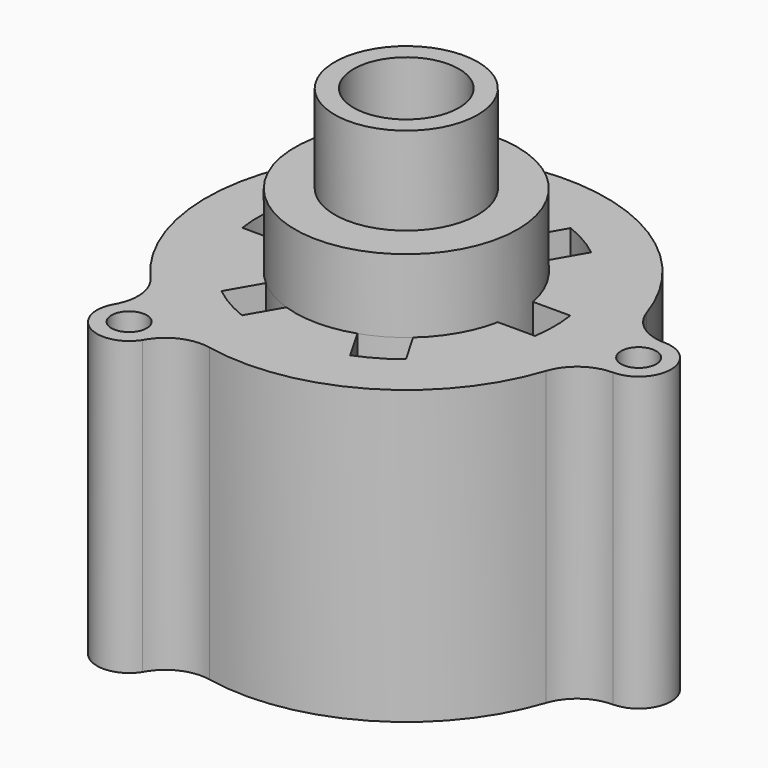
from build123d import *
from build123d import SkipClean  # not in build123d's __all__

# Parameters (mm, degrees)
F0_R      = 7.588
F0_R_2    = 1.105
F1_DEPTH  = 1.32
F2_R      = 7.588
F2_R_2    = 5.588
F3_DEPTH  = 5
F4_R      = 8.638
F4_R_2    = 5.588
F5_DEPTH  = 10
F6_R      = 1.2
F6_R_2    = 3.588
F7_DEPTH  = 2
F8_R      = 1.2
F8_R_2    = 12.138
F9_DEPTH  = 17.92
F10_R     = 4.875
F10_R_2   = 3.588
F11_DEPTH = 11
F13_DEPTH = 2
F15_R     = 7.588
F15_R_2   = 4.875
F16_DEPTH = 5
F17_R     = 5.588
F17_R_2   = 3.588
F18_DEPTH = 13
F19_R     = 7.588
F20_DEPTH = 1.32


# Not quite as in the source:
# - after a boolean that leaves OpenCascade's solid faulty, fix() repairs it


with BuildPart() as f1:
    # F0 (on Top) → F1 (new body)
    with BuildSketch(Plane.XY):
        Circle(F0_R)
        with BuildLine():
            ThreePointArc((-0.0759227724, -1.9785438415), (0.99, -1.7147302995), (1.7514306154, -0.9235208711))
            ThreePointArc((1.7514306154, -0.9235208711), (2.7984444548, -0.5994652894), (3.1225000365, -1.6464791289))
            ThreePointArc((3.1225000365, -1.6464791289), (1.765, -3.0570696754), (-0.1353572659, -3.5274039194))
            ThreePointArc((-0.1353572659, -3.5274039194), (-0.8800700581, -2.7232566337), (-0.0759227724, -1.9785438415))
        make_face(mode=Mode.SUBTRACT)
        with BuildLine():
            ThreePointArc((-2.9871427707, 1.8809247905), (-1.9183743967, 2.1237913442), (-1.675507843, 1.0550229703))
            ThreePointArc((-1.675507843, 1.0550229703), (-1.98, 0), (-1.675507843, -1.0550229703))
            ThreePointArc((-1.675507843, -1.0550229703), (-1.9183743967, -2.1237913442), (-2.9871427707, -1.8809247905))
            ThreePointArc((-2.9871427707, -1.8809247905), (-3.53, 0), (-2.9871427707, 1.8809247905))
        make_face(mode=Mode.SUBTRACT)
        Circle(F0_R_2, mode=Mode.SUBTRACT)
        with BuildLine():
            ThreePointArc((3.1225000365, 1.6464791289), (2.7984444548, 0.5994652894), (1.7514306154, 0.9235208711))
            ThreePointArc((1.7514306154, 0.9235208711), (0.99, 1.7147302995), (-0.0759227724, 1.9785438415))
            ThreePointArc((-0.0759227724, 1.9785438415), (-0.8800700581, 2.7232566337), (-0.1353572659, 3.5274039194))
            ThreePointArc((-0.1353572659, 3.5274039194), (1.765, 3.0570696754), (3.1225000365, 1.6464791289))
        make_face(mode=Mode.SUBTRACT)
    extrude(amount=F1_DEPTH)

    # F2 (on face) → F3 (join)
    with BuildSketch(Plane.XY.offset(1.32)):
        Circle(F2_R)
        Circle(F2_R_2, mode=Mode.SUBTRACT)
    extrude(amount=F3_DEPTH)

    # F4 (on face) → F5 (join)
    with BuildSketch(Plane.XY.offset(6.32)):
        Circle(F4_R)
        Circle(F4_R_2, mode=Mode.SUBTRACT)
    extrude(amount=F5_DEPTH)

    # F6 (on face) → F7 (join)
    with BuildSketch(Plane.XY.offset(16.32)):
        with BuildLine():
            ThreePointArc((-9.7367268731, 12.4452239819), (-9.4590741999, 10.5147410615), (-10.4092493603, 8.8115022416))
            ThreePointArc((-10.4092493603, 8.8115022416), (-13.6367061296, -0.1878561577), (-10.1625749103, -9.0948950073))
            ThreePointArc((-10.1625749103, -9.0948950073), (-9.4051511551, -10.8523580323), (-9.8453718266, -12.7147685106))
            ThreePointArc((-9.8453718266, -12.7147685106), (-9.001992595, -15.6331871577), (-6.0474096405, -14.9268618126))
            ThreePointArc((-6.0474096405, -14.9268618126), (-4.651452375, -13.5895530665), (-2.731783232, -13.361601864))
            ThreePointArc((-2.731783232, -13.361601864), (6.8311346088, -11.8038402208), (12.9462201401, -4.2884062405))
            ThreePointArc((12.9462201401, -4.2884062405), (14.0544760036, -2.7766870908), (15.838, -2.2))
            ThreePointArc((15.838, -2.2), (18.038, 0), (15.838, 2.2))
            ThreePointArc((15.838, 2.2), (14.0544760036, 2.7766870908), (12.9462201401, 4.2884062405))
            ThreePointArc((12.9462201401, 4.2884062405), (6.6468056093, 11.9086111362), (-3.1458537163, 13.2702165919))
            ThreePointArc((-3.1458537163, 13.2702165919), (-4.8713193244, 13.6472554837), (-6.0975711626, 14.9183559205))
            ThreePointArc((-6.0975711626, 14.9183559205), (-9.157320701, 15.5066735299), (-9.7367268731, 12.4452239819))
        make_face()
        with Locations((-7.919, -13.7161103451)):
            Circle(F6_R, mode=Mode.SUBTRACT)
        Circle(F6_R_2, mode=Mode.SUBTRACT)
        with Locations((-7.919, 13.7161103451)):
            Circle(F6_R, mode=Mode.SUBTRACT)
        with Locations((15.838, 0)):
            Circle(F6_R, mode=Mode.SUBTRACT)
    extrude(amount=-F7_DEPTH)

    # F8 (on face) → F9 (join, through all)
    with BuildSketch(Plane(origin=(0, 0, 14.32), x_dir=(1, 0, 0), z_dir=(0, 0, -1))):
        with BuildLine():
            ThreePointArc((-6.0474096405, 14.9268618126), (-9.001992595, 15.6331871577), (-9.8453718266, 12.7147685106))
            ThreePointArc((-9.8453718266, 12.7147685106), (-9.4051511551, 10.8523580323), (-10.1625749103, 9.0948950073))
            ThreePointArc((-10.1625749103, 9.0948950073), (-13.6367061296, 0.1878561577), (-10.4092493603, -8.8115022416))
            ThreePointArc((-10.4092493603, -8.8115022416), (-9.4590741999, -10.5147410615), (-9.7367268731, -12.4452239819))
            ThreePointArc((-9.7367268731, -12.4452239819), (-9.157320701, -15.5066735299), (-6.0975711626, -14.9183559205))
            ThreePointArc((-6.0975711626, -14.9183559205), (-4.8713193244, -13.6472554837), (-3.1458537163, -13.2702165919))
            ThreePointArc((-3.1458537163, -13.2702165919), (6.6468056093, -11.9086111362), (12.9462201401, -4.2884062405))
            ThreePointArc((12.9462201401, -4.2884062405), (14.0544760036, -2.7766870908), (15.838, -2.2))
            ThreePointArc((15.838, -2.2), (18.038, 0), (15.838, 2.2))
            ThreePointArc((15.838, 2.2), (14.0544760036, 2.7766870908), (12.9462201401, 4.2884062405))
            ThreePointArc((12.9462201401, 4.2884062405), (6.8311346088, 11.8038402208), (-2.731783232, 13.361601864))
            ThreePointArc((-2.731783232, 13.361601864), (-4.651452375, 13.5895530665), (-6.0474096405, 14.9268618126))
        make_face()
        with Locations((-7.919, -13.7161103451)):
            Circle(F8_R, mode=Mode.SUBTRACT)
        Circle(F8_R_2, mode=Mode.SUBTRACT)
        with Locations((15.838, 0)):
            Circle(F8_R, mode=Mode.SUBTRACT)
        with Locations((-7.919, 13.7161103451)):
            Circle(F8_R, mode=Mode.SUBTRACT)
    with SkipClean():  # cleaning this boolean's faces spoils the solid; the shape is the same uncleaned
        extrude(amount=F9_DEPTH)

    # F10 (on face) → F11 (join)
    with BuildSketch(Plane.XY.offset(16.32)):
        Circle(F10_R)
        Circle(F10_R_2, mode=Mode.SUBTRACT)
    extrude(amount=F11_DEPTH)

    add(f1.part.fix(), mode=Mode.REPLACE)

    # F12 (on face) → F13 (cut)
    with BuildSketch(Plane.XY.offset(16.32)):
        with BuildLine():
            ThreePointArc((7.4382621626, 1.5), (7.588, 0), (7.4382621626, -1.5))
            Line((7.4382621626, -1.5), (9.9758580583, -1.5))
            ThreePointArc((9.9758580583, -1.5), (10.088, 0), (9.9758580583, 1.5))
            Line((9.9758580583, 1.5), (7.4382621626, 1.5))
        make_face()
        with BuildLine():
            ThreePointArc((2.4200929756, 7.1917239928), (3.794, 6.5714007639), (5.018169187, 5.6917239928))
            Line((5.018169187, 5.6917239928), (6.2869671348, 7.8893465031))
            ThreePointArc((6.2869671348, 7.8893465031), (5.044, 8.7364642734), (3.6888909235, 9.3893465031))
            Line((3.6888909235, 9.3893465031), (2.4200929756, 7.1917239928))
        make_face()
        with BuildLine():
            ThreePointArc((-5.018169187, 5.6917239928), (-3.794, 6.5714007639), (-2.4200929756, 7.1917239928))
            Line((-2.4200929756, 7.1917239928), (-3.6888909235, 9.3893465031))
            ThreePointArc((-3.6888909235, 9.3893465031), (-5.044, 8.7364642734), (-6.2869671348, 7.8893465031))
            Line((-6.2869671348, 7.8893465031), (-5.018169187, 5.6917239928))
        make_face()
        with BuildLine():
            ThreePointArc((-7.4382621626, -1.5), (-7.588, 0), (-7.4382621626, 1.5))
            Line((-7.4382621626, 1.5), (-9.9758580583, 1.5))
            ThreePointArc((-9.9758580583, 1.5), (-10.088, 0), (-9.9758580583, -1.5))
            Line((-9.9758580583, -1.5), (-7.4382621626, -1.5))
        make_face()
        with BuildLine():
            ThreePointArc((-2.4200929756, -7.1917239928), (-3.794, -6.5714007639), (-5.018169187, -5.6917239928))
            Line((-5.018169187, -5.6917239928), (-6.2869671348, -7.8893465031))
            ThreePointArc((-6.2869671348, -7.8893465031), (-5.044, -8.7364642734), (-3.6888909235, -9.3893465031))
            Line((-3.6888909235, -9.3893465031), (-2.4200929756, -7.1917239928))
        make_face()
        with BuildLine():
            ThreePointArc((5.018169187, -5.6917239928), (3.794, -6.5714007639), (2.4200929756, -7.1917239928))
            Line((2.4200929756, -7.1917239928), (3.6888909235, -9.3893465031))
            ThreePointArc((3.6888909235, -9.3893465031), (5.044, -8.7364642734), (6.2869671348, -7.8893465031))
            Line((6.2869671348, -7.8893465031), (5.018169187, -5.6917239928))
        make_face()
    extrude(amount=-F13_DEPTH, mode=Mode.SUBTRACT)

    # F15 (on face) → F16 (join)
    with BuildSketch(Plane.XY.offset(16.32)):
        Circle(F15_R)
        Circle(F15_R_2, mode=Mode.SUBTRACT)
    extrude(amount=F16_DEPTH)

    # F17 (on face) → F18 (join, through all)
    with BuildSketch(Plane.XY.offset(1.32)):
        Circle(F17_R)
        Circle(F17_R_2, mode=Mode.SUBTRACT)
    extrude(amount=F18_DEPTH)

    # F19 (on face) → F20 (cut)
    with BuildSketch(Plane(origin=(0, 0, 0), x_dir=(1, 0, 0), z_dir=(0, 0, -1))):
        Circle(F19_R)
    extrude(amount=-F20_DEPTH, mode=Mode.SUBTRACT)


solid = f1.part
